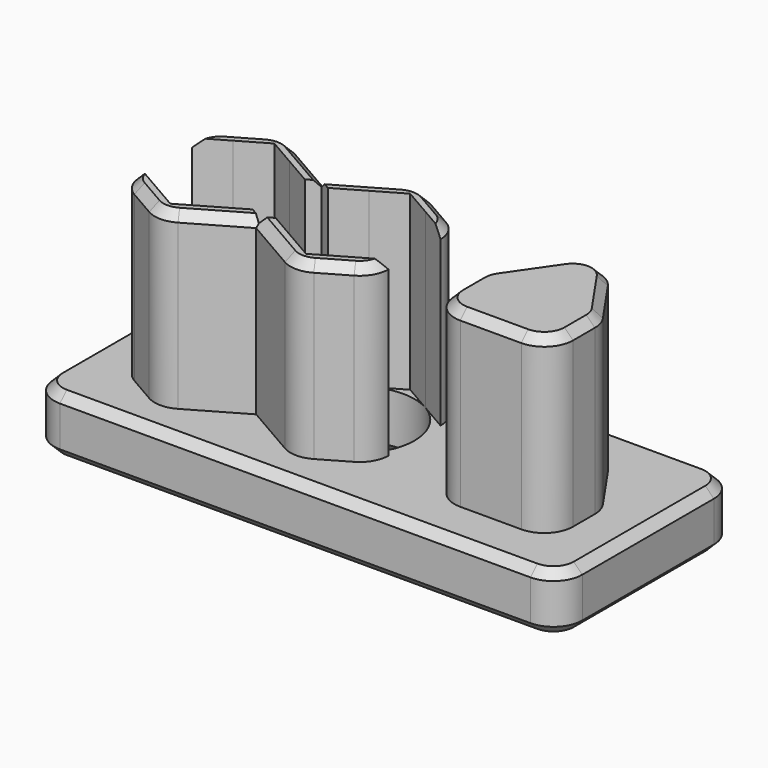
from build123d import *

# Parameters (mm, degrees)
F0_W          = 45.9
F0_H          = 19.3
F0_R          = 4.9
F1_DEPTH      = 5
F3_DEPTH      = 15
F4_T1_DEPTH   = 17.5
F4_T3_DEPTH   = 18.2802116758
F4_T5_DEPTH   = 21.25
F4_T7_DEPTH   = 16.9476143508
F4_T9_DEPTH   = 18.6084391824
F4_T11_DEPTH  = 22.2168783649
F5_T1_DEPTH   = 4.7741809443
F5_T3_DEPTH   = 2.3709542597
F5_T5_DEPTH   = 5.3
F5_T7_DEPTH   = 4.7741809443
F5_T9_DEPTH   = 40.9
F5_T11_DEPTH  = 14.3
F5_T13_DEPTH  = 2.7712812921
F5_T15_DEPTH  = 2.7712812921
F5_T17_DEPTH  = 2.7712812921
F5_T19_DEPTH  = 2.7712812921
F5_T22_ANGLE  = 98.1713551602
F5_T24_ANGLE  = 98.1713551602
F5_T26_ANGLE  = 34.6159793172
F5_T28_ANGLE  = 90.0000000053
F5_T30_ANGLE  = 90.0000000053
F5_T32_ANGLE  = 34.6159793172
F5_T34_ANGLE  = 90.0000000053
F5_T36_ANGLE  = 90.0000000053
F5_T38_ANGLE  = 90.0000000053
F5_T40_ANGLE  = 90.0000000053
F5_T48_DEPTH  = 7.2981197444
F5_T51_ANGLE  = 60.0000000105
F5_T53_ANGLE  = 90.0000000053
F5_T55_ANGLE  = 90.0000000053
F5_T57_ANGLE  = 90.0000000053
F5_T59_ANGLE  = 90.0000000053
F5_T63_DEPTH  = 7.2981197444
F5_T68_DEPTH  = 7.2981197444
F5_T71_ANGLE  = 60.0000000105
F5_T73_ANGLE  = 60.0000000105
F5_T77_DEPTH  = 7.2981197444
F5_T80_ANGLE  = 60.0000000105
F5_T82_ANGLE  = 104.2118652522
F5_T84_ANGLE  = 104.2118652522
F5_T86_ANGLE  = 104.2118652522
F5_T88_ANGLE  = 104.2118652522
F5_T93_DEPTH  = 7.2981197444
F5_T97_DEPTH  = 7.2981197444
F5_T104_DEPTH = 7.2981197444
F5_T108_DEPTH = 7.2981197444


# Not quite as in the source:
# - a fillet or chamfer that OpenCascade refuses, or shapes differently, is made with other operations: its cross-section is extruded or revolved along the edge and cut away or added
# - a feature names something its author has since deleted; it is built from what else it names


with BuildPart() as f1:
    # F0 (on Top) → F1 (new body)
    with BuildSketch(Plane.XY):
        with Locations((2.25, 0)):
            Rectangle(F0_W, F0_H)
        with Locations((-11.8, 0)):
            Circle(F0_R, mode=Mode.SUBTRACT)
        Circle(F0_R, mode=Mode.SUBTRACT)
        Polygon((10.9, 0), (14.8, 5.65), (17.3, 5.65), (21.2, 0), (21.2, -5.65), (10.9, -5.65), align=None, mode=Mode.SUBTRACT)
        Polygon((17.3, 5.65), (14.8, 5.65), (10.9, 0), (10.9, -5.65), (21.2, -5.65), (21.2, 0), align=None)
    extrude(amount=F1_DEPTH)

    # F2 (on face) → F3 (join)
    with BuildSketch(Plane.XY.offset(5)):
        Polygon((14.8, 5.65), (10.9, 0), (10.9, -5.65), (21.2, -5.65), (21.2, 0), (17.3, 5.65), align=None)
        Polygon((-5.65, -3.5507041555), (-5.9, -3.4063665882), (-6.15, -3.5507041555), (-5.9, -3.6950417228), align=None)
        Polygon((-5.9, -3.4063665882), (-6.9, -2.829016319), (-9.3500000593, -4.2435245128), (-11.8, -5.6580326381), (-14.2500001426, -4.2435243962), (-16.7, -2.829016319), (-17.95, -3.5507041555), (-11.8, -7.101408311), (-5.9, -3.6950417228), (-6.15, -3.5507041555), align=None)
        Polygon((-4.9, -2.829016319), (-5.9, -3.4063665882), (-5.65, -3.5507041555), (-5.9, -3.6950417228), (0, -7.101408311), (6.15, -3.5507041555), (4.9, -2.829016319), (2.4499999307, -4.2435245185), (0, -5.6580326381), (-2.4500000255, -4.2435244638), align=None)
        Polygon((-4.9, 2.829016319), (-2.4499999531, 4.2435245056), (0, 5.6580326381), (2.4500000055, 4.2435244754), (4.9, 2.829016319), (6.15, 3.5507041555), (0, 7.101408311), (-5.9, 3.6950417228), (-5.65, 3.5507041555), (-5.9, 3.4063665882), align=None)
        Polygon((-16.7, 2.829016319), (-14.2499999083, 4.2435245315), (-11.8, 5.6580326381), (-9.3500001117, 4.243524543), (-6.9, 2.829016319), (-5.9, 3.4063665882), (-6.15, 3.5507041555), (-5.9, 3.6950417228), (-11.8, 7.101408311), (-17.95, 3.5507041555), align=None)
        Polygon((-6.15, 3.5507041555), (-5.9, 3.4063665882), (-5.65, 3.5507041555), (-5.9, 3.6950417228), align=None)
    extrude(amount=F3_DEPTH)

    # F4: fillet of radius 2.5 on 18 edges, made by hand

    # F4_s2 → F4_t1 (cut)
    with BuildSketch(Plane.XY.offset(-6.25)):
        with BuildLine():
            ThreePointArc((25.2, -7.15), (24.467766953, -8.917766953), (22.7, -9.65))
            Line((22.7, -9.65), (25.2, -9.65))
            Line((25.2, -9.65), (25.2, -7.15))
        make_face()
        with BuildLine():
            ThreePointArc((22.7, 9.65), (24.467766953, 8.917766953), (25.2, 7.15))
            Line((25.2, 7.15), (25.2, 9.65))
            Line((25.2, 9.65), (22.7, 9.65))
        make_face()
        with BuildLine():
            ThreePointArc((-18.2, 9.65), (-19.967766953, 8.917766953), (-20.7, 7.15))
            Line((-20.7, 7.15), (-20.7, 9.65))
            Line((-20.7, 9.65), (-18.2, 9.65))
        make_face()
        with BuildLine():
            ThreePointArc((-20.7, -7.15), (-19.967766953, -8.917766953), (-18.2, -9.65))
            Line((-18.2, -9.65), (-20.7, -9.65))
            Line((-20.7, -9.65), (-20.7, -7.15))
        make_face()
    extrude(amount=F4_T1_DEPTH, mode=Mode.SUBTRACT)

    # F4_s4 → F4_t3 (cut)
    with BuildSketch(Plane.XY.offset(5)):
        with BuildLine():
            ThreePointArc((14.0546397462, 4.570183222), (14.9502882284, 5.3636460935), (16.1120846703, 5.65))
            Line((16.1120846703, 5.65), (14.8, 5.65))
            Line((14.8, 5.65), (14.0546397462, 4.570183222))
        make_face()
        with BuildLine():
            ThreePointArc((18.0453602538, 4.570183222), (17.1497117716, 5.3636460935), (15.9879153297, 5.65))
            Line((15.9879153297, 5.65), (17.3, 5.65))
            Line((17.3, 5.65), (18.0453602538, 4.570183222))
        make_face()
    extrude(amount=F4_T3_DEPTH, mode=Mode.SUBTRACT)

    # F4_s6 → F4_t5 (cut)
    with BuildSketch(Plane.XY.offset(5)):
        with BuildLine():
            ThreePointArc((18.7, -5.65), (20.467766953, -4.917766953), (21.2, -3.15))
            Line((21.2, -3.15), (21.2, -5.65))
            Line((21.2, -5.65), (18.7, -5.65))
        make_face()
        with BuildLine():
            ThreePointArc((10.9, -3.15), (11.632233047, -4.917766953), (13.4, -5.65))
            Line((13.4, -5.65), (10.9, -5.65))
            Line((10.9, -5.65), (10.9, -3.15))
        make_face()
    extrude(amount=F4_T5_DEPTH, mode=Mode.SUBTRACT)

    # F4_s8 → F4_t7 (cut)
    with BuildSketch(Plane.XY.offset(5)):
        with BuildLine():
            ThreePointArc((21.2, -0.7790457403), (21.0867983064, -0.0352757189), (20.7574449242, 0.6411374817))
            Line((20.7574449242, 0.6411374817), (21.2, 0))
            Line((21.2, 0), (21.2, -0.7790457403))
        make_face()
        with BuildLine():
            ThreePointArc((11.3425550758, 0.6411374817), (11.0132016936, -0.0352757189), (10.9, -0.7790457403))
            Line((10.9, -0.7790457403), (10.9, 0))
            Line((10.9, 0), (11.3425550758, 0.6411374817))
        make_face()
    extrude(amount=F4_T7_DEPTH, mode=Mode.SUBTRACT)

    # F4_s10 → F4_t9 (cut)
    with BuildSketch(Plane.XY.offset(5)):
        with BuildLine():
            ThreePointArc((-1.25, -6.3797204745), (0, -6.7146569651), (1.25, -6.3797204745))
            Line((1.25, -6.3797204745), (0, -7.101408311))
            Line((0, -7.101408311), (-1.25, -6.3797204745))
        make_face()
        with BuildLine():
            ThreePointArc((-13.05, -6.3797204745), (-11.8, -6.7146569651), (-10.55, -6.3797204745))
            Line((-10.55, -6.3797204745), (-11.8, -7.101408311))
            Line((-11.8, -7.101408311), (-13.05, -6.3797204745))
        make_face()
        with BuildLine():
            ThreePointArc((1.25, 6.3797204745), (0, 6.7146569651), (-1.25, 6.3797204745))
            Line((-1.25, 6.3797204745), (0, 7.101408311))
            Line((0, 7.101408311), (1.25, 6.3797204745))
        make_face()
        with BuildLine():
            ThreePointArc((-10.55, 6.3797204745), (-11.8, 6.7146569651), (-13.05, 6.3797204745))
            Line((-13.05, 6.3797204745), (-11.8, 7.101408311))
            Line((-11.8, 7.101408311), (-10.55, 6.3797204745))
        make_face()
    extrude(amount=F4_T9_DEPTH, mode=Mode.SUBTRACT)

    # F4_s12 → F4_t11 (cut)
    with BuildSketch(Plane.XY.offset(5)):
        with BuildLine():
            ThreePointArc((4.9, 2.829016319), (4.5650635095, 4.079016319), (3.65, 4.9940798285))
            Line((3.65, 4.9940798285), (6.15, 3.5507041555))
            Line((6.15, 3.5507041555), (4.9, 2.829016319))
        make_face()
        with BuildLine():
            ThreePointArc((3.65, -4.9940798285), (4.5650635095, -4.079016319), (4.9, -2.829016319))
            Line((4.9, -2.829016319), (6.15, -3.5507041555))
            Line((6.15, -3.5507041555), (3.65, -4.9940798285))
        make_face()
        with BuildLine():
            ThreePointArc((-16.7, -2.829016319), (-16.3650635095, -4.079016319), (-15.45, -4.9940798285))
            Line((-15.45, -4.9940798285), (-17.95, -3.5507041555))
            Line((-17.95, -3.5507041555), (-16.7, -2.829016319))
        make_face()
        with BuildLine():
            ThreePointArc((-15.45, 4.9940798285), (-16.3650635095, 4.079016319), (-16.7, 2.829016319))
            Line((-16.7, 2.829016319), (-17.95, 3.5507041555))
            Line((-17.95, 3.5507041555), (-15.45, 4.9940798285))
        make_face()
    extrude(amount=F4_T11_DEPTH, mode=Mode.SUBTRACT)

    # F5: chamfer of 0.75 on 45 edges, made by hand

    # F5_s2 → F5_t1 (cut)
    with BuildSketch(Plane(origin=(6.3988388668, -9.2701127172, 0), x_dir=(0, 0, 1), z_dir=(-0.5680732888, 0.8229779697, 0))):
        Polygon((19.25, 17.4471329569), (20, 16.6971329569), (20, 17.4471329569), align=None)
    extrude(amount=F5_T1_DEPTH, mode=Mode.SUBTRACT)

    # F5_s4 → F5_t3 (cut)
    with BuildSketch(Plane.XZ.offset(0.7790457403)):
        Polygon((21.2, 19.25), (20.45, 20), (21.2, 20), align=None)
        Polygon((10.9, 19.25), (11.65, 20), (10.9, 20), align=None)
    extrude(amount=F5_T3_DEPTH, mode=Mode.SUBTRACT)

    # F5_s6 → F5_t5 (cut)
    with BuildSketch(Plane.YZ.offset(13.4)):
        Polygon((-5.65, 19.25), (-4.9, 20), (-5.65, 20), align=None)
    extrude(amount=F5_T5_DEPTH, mode=Mode.SUBTRACT)

    # F5_s8 → F5_t7 (cut)
    with BuildSketch(Plane(origin=(6.6721488959, 9.666061862, 0), x_dir=(0, 0, 1), z_dir=(-0.5680732888, -0.8229779697, 0))):
        Polygon((19.25, -8.9704598694), (20, -9.7204598694), (20, -8.9704598694), align=None)
    extrude(amount=F5_T7_DEPTH, mode=Mode.SUBTRACT)

    # F5_s10 → F5_t9 (cut)
    with BuildSketch(Plane.YZ.offset(-18.2)):
        Polygon((-8.9, 5), (-9.65, 4.25), (-9.65, 5), align=None)
        Polygon((-8.9, 0), (-9.65, 0.75), (-9.65, 0), align=None)
        Polygon((9.65, 0.75), (8.9, 0), (9.65, 0), align=None)
        Polygon((9.65, 4.25), (8.9, 5), (9.65, 5), align=None)
    extrude(amount=F5_T9_DEPTH, mode=Mode.SUBTRACT)

    # F5_s12 → F5_t11 (cut)
    with BuildSketch(Plane.XZ.offset(-7.15)):
        Polygon((24.45, 0), (25.2, 0.75), (25.2, 0), align=None)
        Polygon((-19.95, 0), (-20.7, 0.75), (-20.7, 0), align=None)
        Polygon((-19.95, 5), (-20.7, 4.25), (-20.7, 5), align=None)
        Polygon((24.45, 5), (25.2, 4.25), (25.2, 5), align=None)
    extrude(amount=F5_T11_DEPTH, mode=Mode.SUBTRACT)

    # F5_s14 → F5_t13 (cut)
    with BuildSketch(Plane(origin=(-1.825, -1.0536642413, 0), x_dir=(0, 0, 1), z_dir=(0.8660254038, 0.5, 0))):
        Polygon((19.25, 6.15), (20, 5.4), (20, 6.15), align=None)
    extrude(amount=F5_T13_DEPTH, mode=Mode.SUBTRACT)

    # F5_s16 → F5_t15 (cut)
    with BuildSketch(Plane(origin=(0.575, -0.3319764048, 0), x_dir=(0, 0, 1), z_dir=(-0.8660254038, 0.5, 0))):
        Polygon((19.25, 6.15), (20, 5.4), (20, 6.15), align=None)
    extrude(amount=F5_T15_DEPTH, mode=Mode.SUBTRACT)

    # F5_s18 → F5_t17 (cut)
    with BuildSketch(Plane(origin=(-7.025, -4.0558856411, 0), x_dir=(0, 0, 1), z_dir=(-0.8660254038, -0.5, 0))):
        Polygon((19.25, 12.05), (20, 11.3), (20, 12.05), align=None)
    extrude(amount=F5_T17_DEPTH, mode=Mode.SUBTRACT)

    # F5_s20 → F5_t19 (cut)
    with BuildSketch(Plane(origin=(-9.425, 5.4415262871, 0), x_dir=(0, 0, 1), z_dir=(0.8660254038, -0.5, 0))):
        Polygon((19.25, 12.05), (20, 11.3), (20, 12.05), align=None)
    extrude(amount=F5_T19_DEPTH, mode=Mode.SUBTRACT)

    # F5_s21 → F5_t22 (revolve, cut)
    with BuildSketch(Plane(origin=(6.6721488969, 9.6660618621, 0), x_dir=(0, 0, 1), z_dir=(-0.5680732888, -0.8229779696, 0))):
        Polygon((19.25, -8.9704598686), (20, -9.7204598686), (20, -8.9704598686), align=None)
    revolve(axis=Axis((16.1120846705, 3.1499999997, 20), (0, 0, -1)), revolution_arc=F5_T22_ANGLE, mode=Mode.SUBTRACT)

    # F5_s23 → F5_t24 (revolve, cut)
    with BuildSketch(Plane(origin=(10.1810745714, 9.4235988418, 0), x_dir=(0, 0, 1), z_dir=(-0.7338800405, -0.6792790929, 0))):
        Polygon((19.25, -6.0485344953), (20, -6.7985344953), (20, -6.0485344953), align=None)
    revolve(axis=Axis((15.9879153295, 3.1499999997, 20), (0, 0, -1)), revolution_arc=F5_T24_ANGLE, mode=Mode.SUBTRACT)

    # F5_s25 → F5_t26 (revolve, cut)
    with BuildSketch(Plane(origin=(6.3988388671, -9.2701127174, 0), x_dir=(0, 0, 1), z_dir=(-0.5680732888, 0.8229779697, 0))):
        Polygon((19.25, 17.4471329568), (20, 16.6971329568), (20, 17.4471329568), align=None)
    revolve(axis=Axis((18.7000000003, -0.7790457401, 20), (0, 0, -1)), revolution_arc=F5_T26_ANGLE, mode=Mode.SUBTRACT)

    # F5_s27 → F5_t28 (revolve, cut)
    with BuildSketch(Plane.XZ.offset(3.1500000001)):
        Polygon((21.2, 19.25), (20.45, 20), (21.2, 20), align=None)
    revolve(axis=Axis((18.7000000001, -3.1500000001, 20), (0, 0, -1)), revolution_arc=F5_T28_ANGLE, mode=Mode.SUBTRACT)

    # F5_s29 → F5_t30 (revolve, cut)
    with BuildSketch(Plane.YZ.offset(13.3999999999)):
        Polygon((-5.65, 19.25), (-4.9, 20), (-5.65, 20), align=None)
    revolve(axis=Axis((13.3999999999, -3.1500000001, 20), (0, 0, -1)), revolution_arc=F5_T30_ANGLE, mode=Mode.SUBTRACT)

    # F5_s31 → F5_t32 (revolve, cut)
    with BuildSketch(Plane.XZ.offset(0.7790457401)):
        Polygon((10.9, 19.25), (11.65, 20), (10.9, 20), align=None)
    revolve(axis=Axis((13.3999999997, -0.7790457401, 20), (0, 0, -1)), revolution_arc=F5_T32_ANGLE, mode=Mode.SUBTRACT)

    # F5_s33 → F5_t34 (revolve, cut)
    with BuildSketch(Plane.YZ.offset(22.7000000001)):
        Polygon((8.9, 0), (9.65, 0.75), (9.65, 0), align=None)
    revolve(axis=Axis((22.7000000001, 7.1500000001, 0), (0, 0, -1)), revolution_arc=F5_T34_ANGLE, mode=Mode.SUBTRACT)

    # F5_s35 → F5_t36 (revolve, cut)
    with BuildSketch(Plane.XZ.offset(7.1500000001)):
        Polygon((24.45, 0), (25.2, 0.75), (25.2, 0), align=None)
    revolve(axis=Axis((22.7000000001, -7.1500000001, 0), (0, 0, -1)), revolution_arc=F5_T36_ANGLE, mode=Mode.SUBTRACT)

    # F5_s37 → F5_t38 (revolve, cut)
    with BuildSketch(Plane.YZ.offset(-18.2000000001)):
        Polygon((-8.9, 0), (-9.65, 0.75), (-9.65, 0), align=None)
    revolve(axis=Axis((-18.2000000001, -7.1500000001, 0), (0, 0, -1)), revolution_arc=F5_T38_ANGLE, mode=Mode.SUBTRACT)

    # F5_s39 → F5_t40 (revolve, cut)
    with BuildSketch(Plane.XZ.offset(-7.1500000001)):
        Polygon((-19.95, 0), (-20.7, 0.75), (-20.7, 0), align=None)
    revolve(axis=Axis((-18.2000000001, 7.1500000001, 0), (0, 0, -1)), revolution_arc=F5_T40_ANGLE, mode=Mode.SUBTRACT)

    # F5_s41 → F5_t42 (revolve, cut)
    with BuildSketch(Plane.XZ):
        Polygon((-6.15, 0), (-6.9, 0.75), (-6.9, 0), align=None)
    revolve(axis=Axis((-11.8, 0, 0), (0, 0, 1)), mode=Mode.SUBTRACT)

    # F5_s43 → F5_t44 (revolve, cut)
    with BuildSketch(Plane.XZ):
        Polygon((5.65, 0), (4.9, 0.75), (4.9, 0), align=None)
    revolve(axis=Axis((0, 0, 0), (0, 0, 1)), mode=Mode.SUBTRACT)


with BuildPart() as f5_tool46:
    # F5_s47 → F5_t48 (new body)
    with BuildSketch(Plane(origin=(-10.675, -6.1632141236, 0), x_dir=(0, 0, 1), z_dir=(0.8660254038, 0.5, 0))):
        Polygon((19.25, 0.25), (20, -0.5), (20, 0.25), align=None)
    extrude(amount=F5_T48_DEPTH)

    split(bisect_by=Plane(origin=(-3.075, -5.3260562333, 0), x_dir=(0, 0, 1), z_dir=(-0.5, -0.8660254038, 0)), keep=Keep.TOP)


with BuildPart() as f1_1:
    add(f1.part)

    # F5_t45: cut F5_tool46
    add(f5_tool46.part, mode=Mode.SUBTRACT)

    # F5_s50 → F5_t51 (revolve, cut)
    with BuildSketch(Plane(origin=(-7.0249999987, -4.0558856412, 0), x_dir=(0, 0, 1), z_dir=(-0.8660254037, -0.5000000001, 0))):
        Polygon((19.25, 12.0500000007), (20, 11.3000000007), (20, 12.0500000007), align=None)
    revolve(axis=Axis((-11.8, 4.2146569655, 20), (0, 0, -1)), revolution_arc=F5_T51_ANGLE, mode=Mode.SUBTRACT)

    # F5_s52 → F5_t53 (revolve, cut)
    with BuildSketch(Plane.XZ.offset(-7.1500000001)):
        Polygon((-20.7, 4.25), (-19.95, 5), (-20.7, 5), align=None)
    revolve(axis=Axis((-18.2000000001, 7.1500000001, 5), (0, 0, -1)), revolution_arc=F5_T53_ANGLE, mode=Mode.SUBTRACT)

    # F5_s54 → F5_t55 (revolve, cut)
    with BuildSketch(Plane.YZ.offset(22.7000000001)):
        Polygon((8.9, 5), (9.65, 4.25), (9.65, 5), align=None)
    revolve(axis=Axis((22.7000000001, 7.1500000001, 5), (0, 0, -1)), revolution_arc=F5_T55_ANGLE, mode=Mode.SUBTRACT)

    # F5_s56 → F5_t57 (revolve, cut)
    with BuildSketch(Plane.YZ.offset(-18.2000000001)):
        Polygon((-8.9, 5), (-9.65, 4.25), (-9.65, 5), align=None)
    revolve(axis=Axis((-18.2000000001, -7.1500000001, 5), (0, 0, -1)), revolution_arc=F5_T57_ANGLE, mode=Mode.SUBTRACT)

    # F5_s58 → F5_t59 (revolve, cut)
    with BuildSketch(Plane.XZ.offset(7.1500000001)):
        Polygon((24.45, 5), (25.2, 4.25), (25.2, 5), align=None)
    revolve(axis=Axis((22.7000000001, -7.1500000001, 5), (0, 0, -1)), revolution_arc=F5_T59_ANGLE, mode=Mode.SUBTRACT)


with BuildPart() as f5_tool61:
    # F5_s62 → F5_t63 (new body)
    with BuildSketch(Plane(origin=(-4.3546429015, 2.5141542514, 0), x_dir=(0, 0, 1), z_dir=(-0.8660254038, 0.5, 0))):
        Polygon((19.25, 0.25), (20, -0.5), (20, 0.25), align=None)
    extrude(amount=F5_T63_DEPTH)

    split(bisect_by=Plane(origin=(-3.075, 5.3260562333, 0), x_dir=(0, 0, 1), z_dir=(-0.5, 0.8660254038, 0)), keep=Keep.TOP)


with BuildPart() as f1_2:
    add(f1_1.part)

    # F5_t60: cut F5_tool61
    add(f5_tool61.part, mode=Mode.SUBTRACT)


with BuildPart() as f5_tool66:
    # F5_s67 → F5_t68 (new body)
    with BuildSketch(Plane(origin=(1.825, 1.0536642413, 0), x_dir=(0, 0, 1), z_dir=(-0.8660254038, -0.5, 0))):
        Polygon((19.25, 6.15), (20, 5.4), (20, 6.15), align=None)
    extrude(amount=F5_T68_DEPTH)

    split(bisect_by=Plane(origin=(0.125, 0.2165063509, 0), x_dir=(0, 0, 1), z_dir=(0.5, 0.8660254038, 0)), keep=Keep.TOP)


with BuildPart() as f1_3:
    add(f1_2.part)

    # F5_t65: cut F5_tool66
    add(f5_tool66.part, mode=Mode.SUBTRACT)

    # F5_s70 → F5_t71 (revolve, cut)
    with BuildSketch(Plane(origin=(1.8250000004, 1.0536642417, 0), x_dir=(0, 0, 1), z_dir=(-0.8660254037, -0.5000000001, 0))):
        Polygon((19.25, 6.1499999998), (20, 5.3999999998), (20, 6.1499999998), align=None)
    revolve(axis=Axis((0, 4.2146569655, 20), (0, 0, -1)), revolution_arc=F5_T71_ANGLE, mode=Mode.SUBTRACT)

    # F5_s72 → F5_t73 (revolve, cut)
    with BuildSketch(Plane(origin=(-1.8250000004, -1.0536642417, 0), x_dir=(0, 0, 1), z_dir=(0.8660254037, 0.5000000001, 0))):
        Polygon((19.25, 6.1499999998), (20, 5.3999999998), (20, 6.1499999998), align=None)
    revolve(axis=Axis((0, -4.2146569655, 20), (0, 0, -1)), revolution_arc=F5_T73_ANGLE, mode=Mode.SUBTRACT)


with BuildPart() as f5_tool75:
    # F5_s76 → F5_t77 (new body)
    with BuildSketch(Plane(origin=(-4.4953570985, 2.5953956309, 0), x_dir=(0, 0, 1), z_dir=(0.8660254038, -0.5, 0))):
        Polygon((19.25, 6.15), (20, 5.4), (20, 6.15), align=None)
    extrude(amount=F5_T77_DEPTH)

    split(bisect_by=Plane(origin=(0.125, -0.2165063509, 0), x_dir=(0, 0, 1), z_dir=(0.5, -0.8660254038, 0)), keep=Keep.TOP)


with BuildPart() as f1_4:
    add(f1_3.part)

    # F5_t74: cut F5_tool75
    add(f5_tool75.part, mode=Mode.SUBTRACT)

    # F5_s79 → F5_t80 (revolve, cut)
    with BuildSketch(Plane(origin=(-10.6749999994, -6.1632141246, 0), x_dir=(0, 0, 1), z_dir=(0.8660254037, 0.5000000001, 0))):
        Polygon((19.25, 0.2499999988), (20, -0.5000000012), (20, 0.2499999988), align=None)
    revolve(axis=Axis((-11.8, -4.2146569655, 20), (0, 0, -1)), revolution_arc=F5_T80_ANGLE, mode=Mode.SUBTRACT)

    # F5_s81 → F5_t82 (revolve, cut)
    with BuildSketch(Plane(origin=(-8.3186687816, 8.5507312317, 0), x_dir=(0, 0, 1), z_dir=(0.6973135513, -0.716766218, 0))):
        Polygon((19.25, 10.705368879), (20, 9.955368879), (20, 10.705368879), align=None)
    revolve(axis=Axis((-14.2000000001, 2.8290163191, 20), (0, 0, -1)), revolution_arc=F5_T82_ANGLE, mode=Mode.SUBTRACT)

    # F5_s83 → F5_t84 (revolve, cut)
    with BuildSketch(Plane(origin=(0.5750000001, -0.3319764048, 0), x_dir=(0, 0, 1), z_dir=(-0.8660254038, 0.5, 0))):
        Polygon((20, 5.4), (19.25, 6.15), (20, 6.15), align=None)
    revolve(axis=Axis((2.4000000001, 2.8290163191, 20), (0, 0, -1)), revolution_arc=F5_T84_ANGLE, mode=Mode.SUBTRACT)

    # F5_s85 → F5_t86 (revolve, cut)
    with BuildSketch(Plane(origin=(2.580963754, -2.6529638285, 0), x_dir=(0, 0, 1), z_dir=(-0.6973135513, 0.716766218, 0))):
        Polygon((19.25, 2.247527507), (20, 1.497527507), (20, 2.247527507), align=None)
    revolve(axis=Axis((2.4000000001, -2.8290163191, 20), (0, 0, -1)), revolution_arc=F5_T86_ANGLE, mode=Mode.SUBTRACT)

    # F5_s87 → F5_t88 (revolve, cut)
    with BuildSketch(Plane(origin=(-9.4250000003, 5.441526287, 0), x_dir=(0, 0, 1), z_dir=(0.8660254038, -0.5, 0))):
        Polygon((20, 11.2999999998), (19.25, 12.0499999998), (20, 12.0499999998), align=None)
    revolve(axis=Axis((-14.2000000001, -2.8290163191, 20), (0, 0, -1)), revolution_arc=F5_T88_ANGLE, mode=Mode.SUBTRACT)


with BuildPart() as f5_tool91:
    # F5_s92 → F5_t93 (new body)
    with BuildSketch(Plane(origin=(-4.4953570985, 2.5953956309, 0), x_dir=(0, 0, 1), z_dir=(0.8660254038, -0.5, 0))):
        Polygon((19.25, 6.15), (20, 5.4), (20, 6.15), align=None)
    extrude(amount=F5_T93_DEPTH)

    split(bisect_by=Plane(origin=(0.125, -0.2165063509, 0), x_dir=(0, 0, 1), z_dir=(-0.5, 0.8660254038, 0)), keep=Keep.TOP)


with BuildPart() as f5_tool95:
    # F5_s96 → F5_t97 (new body)
    with BuildSketch(Plane(origin=(-10.675, -6.1632141236, 0), x_dir=(0, 0, 1), z_dir=(0.8660254038, 0.5, 0))):
        Polygon((19.25, 0.25), (20, -0.5), (20, 0.25), align=None)
    extrude(amount=F5_T97_DEPTH)

    split(bisect_by=Plane(origin=(-3.075, -5.3260562333, 0), x_dir=(0, 0, 1), z_dir=(0.5, 0.8660254038, 0)), keep=Keep.TOP)


with BuildPart() as f5_tool91_1:
    add(f5_tool91.part)

    # F5_t99: intersect F5_tool95
    add(f5_tool95.part, mode=Mode.INTERSECT)


with BuildPart() as f1_5:
    add(f1_4.part)

    # F5_t89: cut F5_tool91
    add(f5_tool91_1.part, mode=Mode.SUBTRACT)


with BuildPart() as f5_tool102:
    # F5_s103 → F5_t104 (new body)
    with BuildSketch(Plane(origin=(-4.3546429015, 2.5141542514, 0), x_dir=(0, 0, 1), z_dir=(-0.8660254038, 0.5, 0))):
        Polygon((19.25, 0.25), (20, -0.5), (20, 0.25), align=None)
    extrude(amount=F5_T104_DEPTH)

    split(bisect_by=Plane(origin=(-3.075, 5.3260562333, 0), x_dir=(0, 0, 1), z_dir=(0.5, -0.8660254038, 0)), keep=Keep.TOP)


with BuildPart() as f5_tool106:
    # F5_s107 → F5_t108 (new body)
    with BuildSketch(Plane(origin=(1.825, 1.0536642413, 0), x_dir=(0, 0, 1), z_dir=(-0.8660254038, -0.5, 0))):
        Polygon((19.25, 6.15), (20, 5.4), (20, 6.15), align=None)
    extrude(amount=F5_T108_DEPTH)

    split(bisect_by=Plane(origin=(0.125, 0.2165063509, 0), x_dir=(0, 0, 1), z_dir=(-0.5, -0.8660254038, 0)), keep=Keep.TOP)


with BuildPart() as f5_tool102_1:
    add(f5_tool102.part)

    # F5_t110: intersect F5_tool106
    add(f5_tool106.part, mode=Mode.INTERSECT)


with BuildPart() as f1_6:
    add(f1_5.part)

    # F5_t100: cut F5_tool102
    add(f5_tool102_1.part, mode=Mode.SUBTRACT)


solid = f1_6.part
